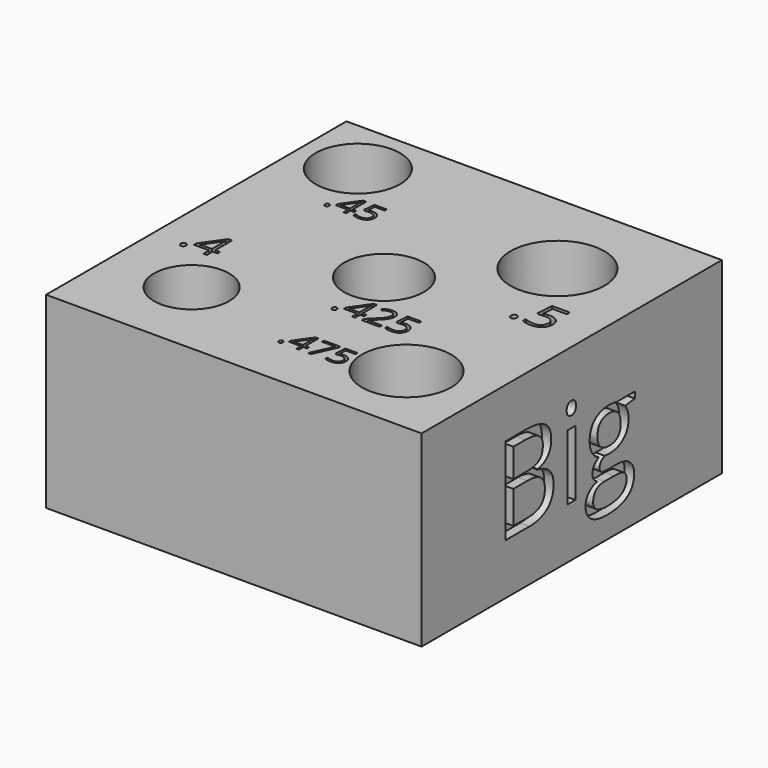
from build123d import *

# Parameters (mm, degrees)
F0_W           = 50.8
F0_H           = 50.8
F1_DEPTH       = 25.4
F2_R           = 6.0325
F2_R_2         = 5.08
F2_R_3         = 5.715
F2_R_4         = 6.35
F2_R_5         = 5.3975
F3_DEPTH       = 12.7
F2_TEXT_SIZE   = 6.6860734175
F2_TEXT_SIZE_2 = 4.5728843866
F2_TEXT_SIZE_3 = 5.9178487087
F2_TEXT_SIZE_4 = 4.7544941553
F4_DEPTH       = 1.27
F5_TEXT_SIZE   = 5.168275274
F6_DEPTH       = 1.27
F7_TEXT_SIZE   = 16.5101580529
F8_DEPTH       = 1.27


# Not quite as in the source:
# - Text() gives the source's letters only with a copy of the font that has no kerning and outlines rounded to 1/6400 em; it was checked with that copy


with BuildPart() as f1:
    # F0 (on Top) → F1 (new body)
    with BuildSketch(Plane.XY):
        Rectangle(F0_W, F0_H)
    extrude(amount=F1_DEPTH)

    # F2 (on face) → F3 (cut)
    with BuildSketch(Plane.XY.offset(25.4)):
        with Locations((15.2345848073, -15.2345848073)):
            Circle(F2_R)
        with Locations((-14.4618223182, -14.4618223182)):
            Circle(F2_R_2)
        with Locations((-17.7022340127, 17.7022340127)):
            Circle(F2_R_3)
        with Locations((13.0363431647, 13.0363431647)):
            Circle(F2_R_4)
        Circle(F2_R_5)
    extrude(amount=-F3_DEPTH, mode=Mode.SUBTRACT)

    # F2 (on face) → F4 (cut)
    with BuildSketch(Plane.XY.offset(25.4)):
        with Locations((15.4480698984, 1.2136949226)):
            Text('.5', F2_TEXT_SIZE, font='Open Sans', text_align=(TextAlign.LEFT, TextAlign.BOTTOM))
        with Locations((0.0648610294, -18.5270615657)):
            Text('.475', F2_TEXT_SIZE_2, font='Open Sans', text_align=(TextAlign.LEFT, TextAlign.BOTTOM))
        with Locations((-22.0207097009, -7.6862764545)):
            Text('.4', F2_TEXT_SIZE_3, font='Open Sans', text_align=(TextAlign.LEFT, TextAlign.BOTTOM))
        with Locations((-15.6729395236, 8.9364156173)):
            Text('.45', F2_TEXT_SIZE_4, font='Open Sans', text_align=(TextAlign.LEFT, TextAlign.BOTTOM))
    extrude(amount=-F4_DEPTH, mode=Mode.SUBTRACT)

    # F5 (on face) → F6 (cut)
    with BuildSketch(Plane.XY.offset(25.4)):
        with Locations((-0.304956617, -9.1100363469)):
            Text('.425', F5_TEXT_SIZE, font='Open Sans', text_align=(TextAlign.LEFT, TextAlign.BOTTOM))
    extrude(amount=-F6_DEPTH, mode=Mode.SUBTRACT)

    # F7 (on face) → F8 (cut)
    with BuildSketch(Plane.YZ.offset(25.4)):
        with Locations((-12.8569421358, 6.9014914334)):
            Text('Big', F7_TEXT_SIZE, font='Open Sans', text_align=(TextAlign.LEFT, TextAlign.BOTTOM))
    extrude(amount=-F8_DEPTH, mode=Mode.SUBTRACT)


solid = f1.part
